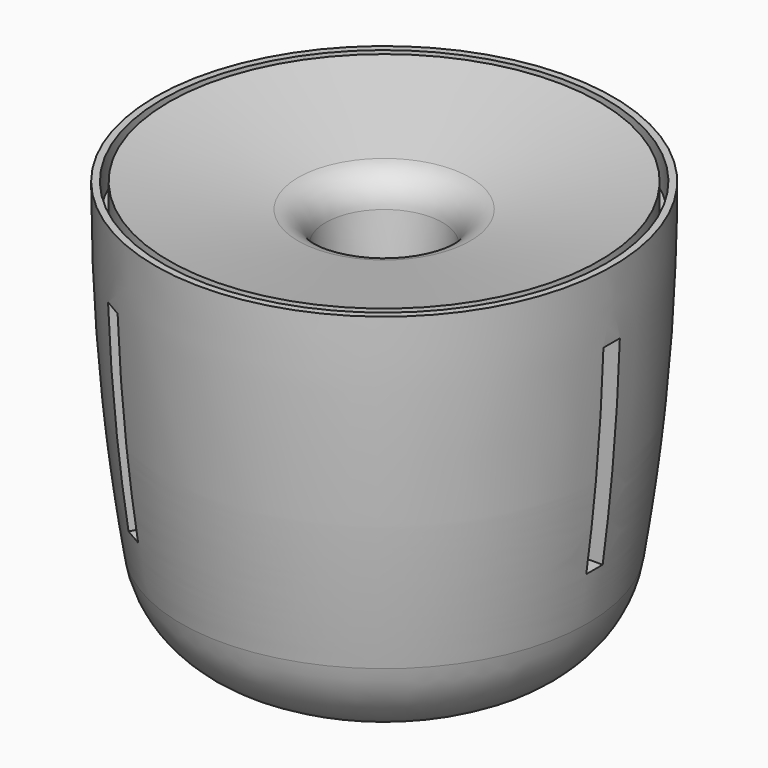
from build123d import *

# Parameters (mm, degrees)
F3_DEPTH         = 11.5
F5_R             = 8
F6_DEPTH         = 25
F7_R             = 0.5
F8_R             = 2
F9_R             = 1
F11_DEPTH        = 1.5
F11_COPIES_COUNT = 3


# Not quite as in the source:
# - a pattern or mirror of a feature is missing from the dataset's text; its kind, count and spacing are read off the source's solid


with BuildPart() as f1:
    # F0 (on Front) → F1 (revolve)
    with BuildSketch(Plane.XZ):
        with BuildLine():
            Line((-12.5923461222, 23.0231059935), (-31.5, 26.6159944863))
            Line((-31.5, 26.6159944863), (-31.5, 21.6159944863))
            Line((-31.5, 21.6159944863), (-32.5, 21.6159944863))
            Line((-32.5, 21.6159944863), (-32.5, 26.6159944863))
            Line((-32.5, 26.6159944863), (-33.5, 26.6159944863))
            ThreePointArc((-33.5, 26.6159944863), (-32.559738199, 2.8826216042), (-29.7448467442, -20.7019807185))
            ThreePointArc((-29.7448467442, -20.7019807185), (-24.647599638, -29.7828571781), (-14.876418747, -33.3840055137))
            Line((-14.876418747, -33.3840055137), (-7.5, -33.3840055137))
            Line((-7.5, -33.3840055137), (-7.5, 5.7419622669))
            ThreePointArc((-7.5, 5.7419622669), (-7.5190709956, 6.6151610531), (-7.576247612, 7.4866945623))
            Line((-7.576247612, 7.4866945623), (-8.5448201406, 18.5471874985))
            ThreePointArc((-8.5448201406, 18.5471874985), (-9.8172078197, 21.4646075314), (-12.5923461222, 23.0231059935))
        make_face()
    revolve(axis=Axis((0, 0, 3.0846800655), (0, 0, 1)))

    # F2 (on Front) → F3 (cut, symmetric)
    with BuildSketch(Plane.XZ):
        Polygon((26, 3.7419622669), (-23.5, 3.7419622669), (-23.5, -21.7580377331), (26, -21.7580377331), (26, -18.2580377331), (-11, -18.2580377331), (-11, 0.2419622669), (26, 0.2419622669), align=None)
    extrude(amount=F3_DEPTH, both=True, mode=Mode.SUBTRACT)

    # F5 (on offset) → F6 (cut)
    with BuildSketch(Plane.YZ.offset(-18)):
        with Locations((0, -9.2580377331)):
            Circle(F5_R)
    extrude(amount=-F6_DEPTH, mode=Mode.SUBTRACT)

    # F7
    f7_edges = [f1.edges().sort_by_distance(p)[0] for p in [
        (-30.318545, -7.999666, -9.184947),
        (-30.084057, 5.659565, -14.91218),
        (-31.464589, 5.675758, -3.620151),
    ]]
    fillet(f7_edges, radius=F7_R)

    # F8
    f8_edges = [f1.edges().sort_by_distance(p)[0] for p in [
        (7.5, 0, -33.384006),
    ]]
    fillet(f8_edges, radius=F8_R)

    # F9
    f9_edges = [f1.edges().sort_by_distance(p)[0] for p in [
        (7.5, 0, -21.758038),
        (7.5, 0, -18.258038),
        (7.5, 0, 0.241962),
        (7.5, 0, 3.741962),
        (-11, 0, 0.241962),
        (-11, 0, -18.258038),
    ]]
    fillet(f9_edges, radius=F9_R)

    # F10 (on Front) → F11 (cut, symmetric)
    with BuildSketch(Plane.XZ):
        with BuildLine():
            Line((28.3332870113, -13.3840055137), (30.8213749464, -13.3840055137))
            ThreePointArc((30.8213749464, -13.3840055137), (32.4538803469, 1.5844658563), (33.3332870113, 16.6159944863))
            Line((33.3332870113, 16.6159944863), (28.3332870113, 16.6159944863))
            Line((28.3332870113, 16.6159944863), (28.3332870113, -13.3840055137))
        make_face()
    f11 = extrude(amount=F11_DEPTH, both=True, mode=Mode.SUBTRACT)

    # F11_copies: F11 ×3 about axis
    f11_copies_axis = Axis((0, 0, 0), (0, 0, 1))
    for i in range(1, F11_COPIES_COUNT):
        add(f11.rotate(f11_copies_axis, i * 360 / F11_COPIES_COUNT), mode=Mode.SUBTRACT)


solid = f1.part
